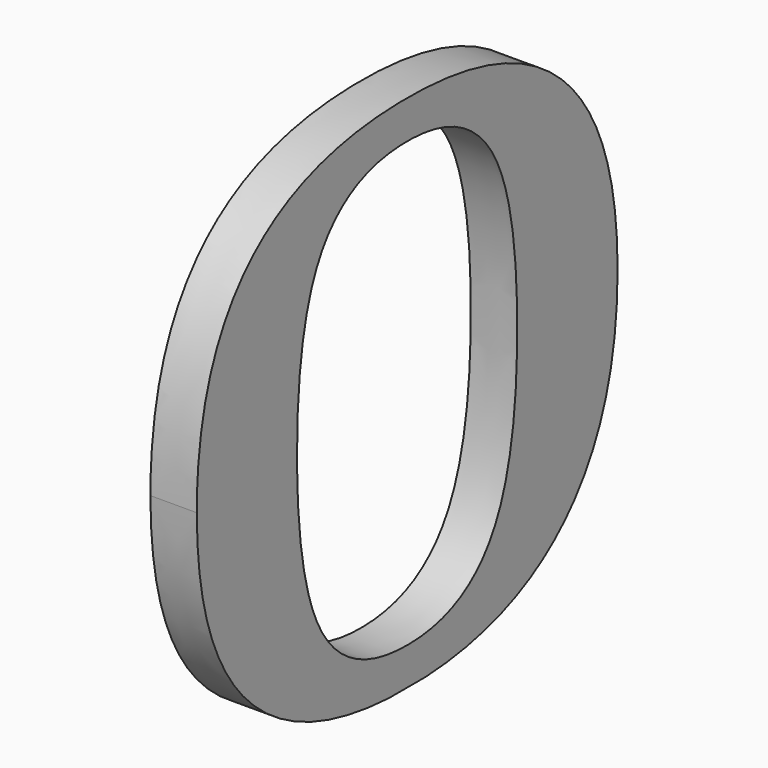
from build123d import *

# Parameters (mm, degrees)
F0_TEXT_SIZE = 635
F1_DEPTH     = 38.1
F2_W         = 133.3039700985
F2_H         = 5.8454149403
F3_DEPTH     = 38.1010001


# Not quite as in the source:
# - Text() gives the source's letters only with a copy of the font that has no kerning and outlines rounded to 1/6400 em; it was checked with that copy


with BuildPart() as f1:
    # F0 (on Right) → F1 (new body)
    with BuildSketch(Plane.YZ):
        with Locations((-502.6421875, 0)):
            Text('O', F0_TEXT_SIZE, font='Tinos', font_style=FontStyle.BOLD, text_align=(TextAlign.LEFT, TextAlign.BOTTOM))
    extrude(amount=F1_DEPTH)

    # F2 (on face) → F3 (cut, through all)
    with BuildSketch(Plane.YZ.offset(38.1)):
        with Locations((-250.3666132689, -8.7158109527)):
            Rectangle(F2_W, F2_H)
    extrude(amount=-F3_DEPTH, mode=Mode.SUBTRACT)


solid = f1.part
